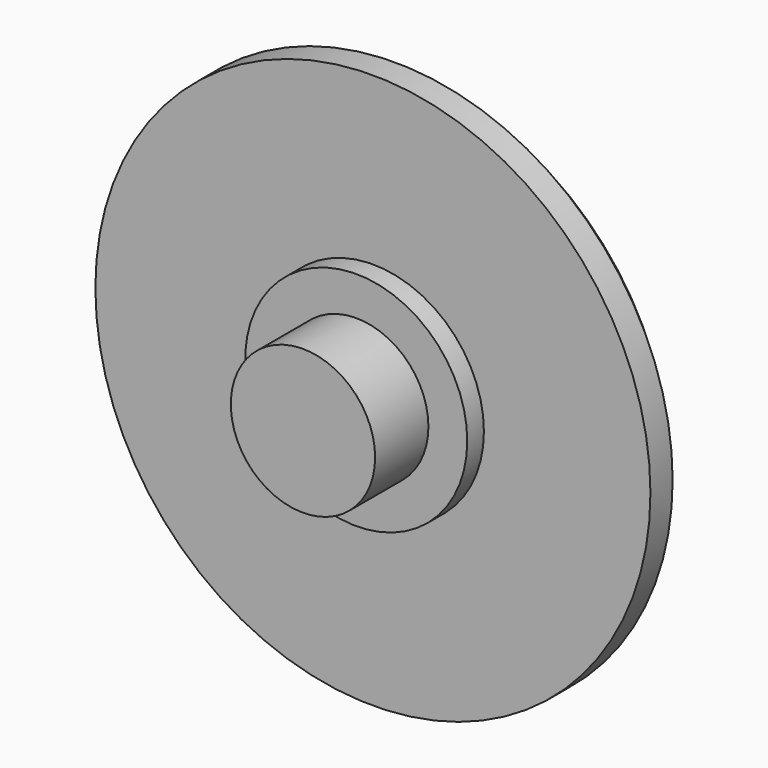
from build123d import *

# Parameters (mm, degrees)
F2_R        = 2.5
F3_DEPTH    = 1.5
F4_R        = 1
F5_S5_R     = 2.5
F5_T6_DEPTH = 16


# Not quite as in the source:
# - a fillet or chamfer that OpenCascade refuses, or shapes differently, is made with other operations: its cross-section is extruded or revolved along the edge and cut away or added


with BuildPart() as f1:
    # F0 (on Top) → F1 (revolve)
    with BuildSketch(Plane.XY):
        Polygon((0, 0), (0, -4.9), (2.6, -4.9), (2.6, -2.8), (2.6, -2.5), (4, -2.5), (4, -1.75), (10, -1.75), (10, 0), align=None)
    revolve(axis=Axis((0, -2.45, 0), (0, -1, 0)))

    # F2 (on face) → F3 (join)
    with BuildSketch(Plane(origin=(0, 0, 0), x_dir=(-1, 0, 0), z_dir=(0, 1, 0))):
        with Locations((7, 0)):
            Circle(F2_R)
    extrude(amount=F3_DEPTH)

    # F4
    f4_edges = [f1.edges().sort_by_distance(p)[0] for p in [
        (-4.5, 1.5, 0),
    ]]
    fillet(f4_edges, radius=F4_R)

    # F5: chamfer of 0.75 on 1 edges, made by hand


with BuildPart() as f5_tool2:
    # F5_s3 → F5_t4 (revolve)
    with BuildSketch(Plane.XY):
        Polygon((9.25, 0), (10, -0.75), (10, 0), align=None)
    revolve(axis=Axis((0, 0, 0), (0, -1, 0)))

    # F5_s5 → F5_t6 (cut, symmetric)
    with BuildSketch(Plane.XZ.offset(0.4)):
        with Locations((-7, 0)):
            Circle(F5_S5_R)
    extrude(amount=F5_T6_DEPTH, both=True, mode=Mode.SUBTRACT)


with BuildPart() as f1_1:
    add(f1.part)

    # F5_t1: cut F5_tool2
    add(f5_tool2.part, mode=Mode.SUBTRACT)


solid = f1_1.part
